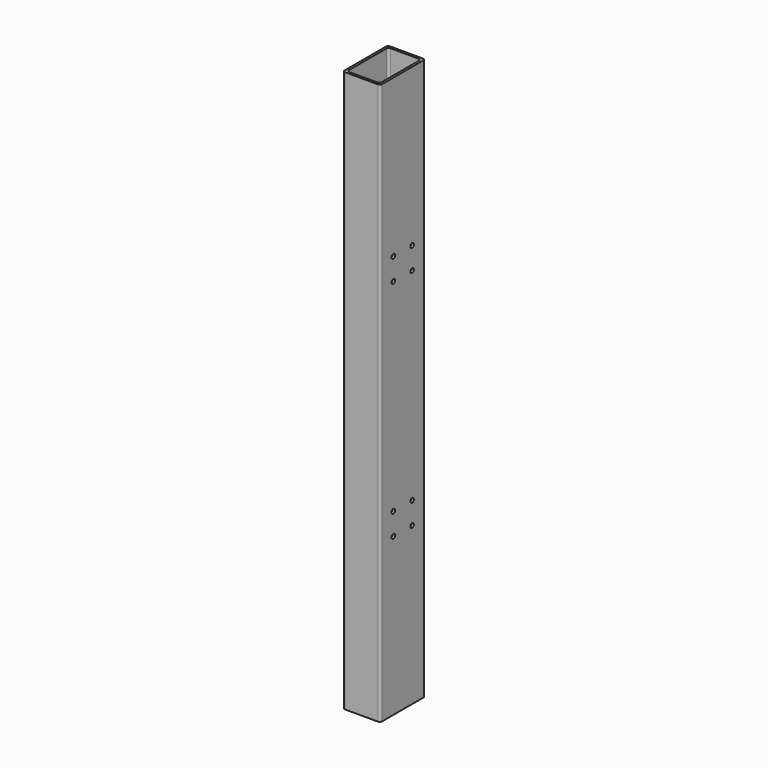
from build123d import *

# Parameters (mm, degrees)
F0_W     = 50.8
F0_H     = 76.2
F0_W_2   = 44.45
F0_H_2   = 69.85
F2_DEPTH = 762
F3_R     = 3.175
F4_R     = 3
F5_DEPTH = 50.801
F6_W     = 69.85
F6_H     = 379.5014
F6_R     = 3
F7_DEPTH = 25.4


# Not quite as in the source:
# - a variable given as a bare number and used for a length is read in inches; the dataset says mm whatever the document's units were


with BuildPart() as f2:
    # F0 (on Top) → F2 (new body)
    with BuildSketch(Plane.XY):
        Rectangle(F0_W, F0_H)
        Rectangle(F0_W_2, F0_H_2, mode=Mode.SUBTRACT)
    extrude(amount=F2_DEPTH)

    # F3
    f3_edges = [f2.edges().sort_by_distance(p)[0] for p in [
        (-22.225, 34.925, 381),
        (22.225, 34.925, 381),
        (22.225, -34.925, 381),
        (-22.225, -34.925, 381),
        (25.4, 38.1, 381),
        (-25.4, 38.1, 381),
        (25.4, -38.1, 381),
        (-25.4, -38.1, 381),
    ]]
    fillet(f3_edges, radius=F3_R)

    # F4 (on face) → F5 (cut, through all)
    with BuildSketch(Plane.YZ.offset(25.4)):
        with Locations((-16, 213.6)):
            Circle(F4_R)
        with Locations((-16, 243.6)):
            Circle(F4_R)
        with Locations((16, 243.6)):
            Circle(F4_R)
        with Locations((16, 213.6)):
            Circle(F4_R)
        with Locations((-16, 518.4)):
            Circle(F4_R)
        with Locations((-16, 548.4)):
            Circle(F4_R)
        with Locations((16, 518.4)):
            Circle(F4_R)
        with Locations((16, 548.4)):
            Circle(F4_R)
    extrude(amount=-F5_DEPTH, mode=Mode.SUBTRACT)

    # F6 (on face) → F7 (cut)
    with BuildSketch(Plane(origin=(-25.4, 0, 0), x_dir=(0, -1, 0), z_dir=(-1, 0, 0))):
        with Locations((0, 382.9008626968)):
            Rectangle(F6_W, F6_H)
        with Locations((-16, 213.6)):
            Circle(F6_R, mode=Mode.SUBTRACT)
        with Locations((-16, 243.6)):
            Circle(F6_R, mode=Mode.SUBTRACT)
        with Locations((16, 213.6)):
            Circle(F6_R, mode=Mode.SUBTRACT)
        with Locations((16, 243.6)):
            Circle(F6_R, mode=Mode.SUBTRACT)
        with Locations((-16, 518.4)):
            Circle(F6_R, mode=Mode.SUBTRACT)
        with Locations((-16, 548.4)):
            Circle(F6_R, mode=Mode.SUBTRACT)
        with Locations((16, 518.4)):
            Circle(F6_R, mode=Mode.SUBTRACT)
        with Locations((16, 548.4)):
            Circle(F6_R, mode=Mode.SUBTRACT)
    extrude(amount=-F7_DEPTH, mode=Mode.SUBTRACT)


solid = f2.part
